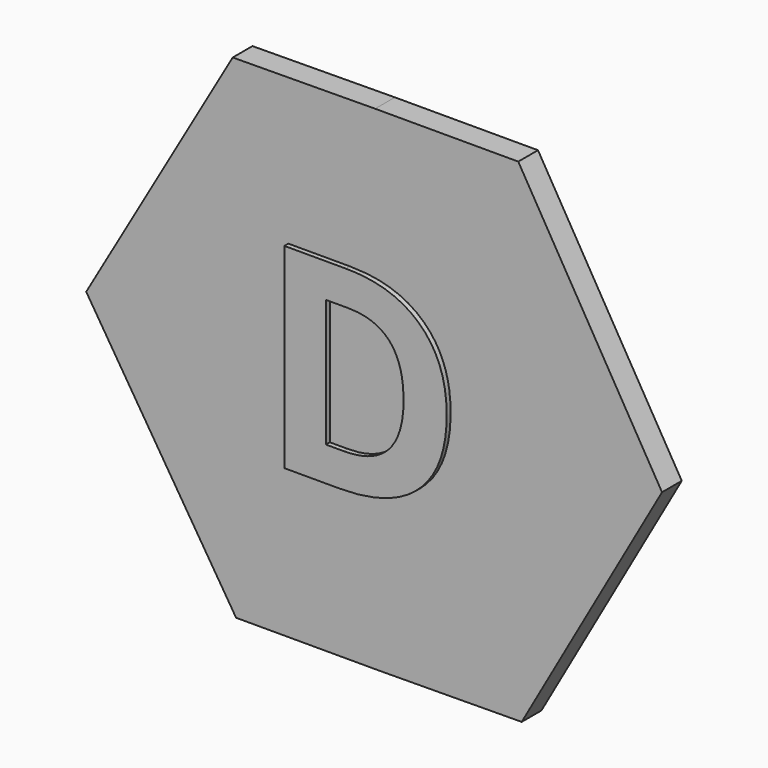
from build123d import *

# Parameters (mm, degrees)
F1_TEXT_SIZE = 35.2777777778
F2_DEPTH     = 3.81
F3_DEPTH     = 3.175


# Not quite as in the source:
# - Text() gives the source's letters only with a copy of the font that has no kerning and outlines rounded to 1/6400 em; it was checked with that copy


with BuildPart() as f2:
    # F1 (on Front) → F2 (new body)
    with BuildSketch(Plane.XZ):
        with Locations((-14.6136979561, -12.3520550598)):
            Text('D', F1_TEXT_SIZE, font='Open Sans', font_style=FontStyle.BOLD, text_align=(TextAlign.LEFT, TextAlign.BOTTOM))
    extrude(amount=F2_DEPTH)

    # F0 (on Front) → F3 (join)
    with BuildSketch(Plane.XZ):
        Polygon((36.6617420935, 0.3062387457), (18.1557776481, 31.75), (-0.2652105334, 31.75), (-18.5960815801, 31.5968806272), (-37.4514907598, -1.0833075503), (-18.1619734366, -31.75), (0.2652105333, -31.75), (18.5960815801, -31.5968806272), align=None)
    extrude(amount=F3_DEPTH)


solid = f2.part
